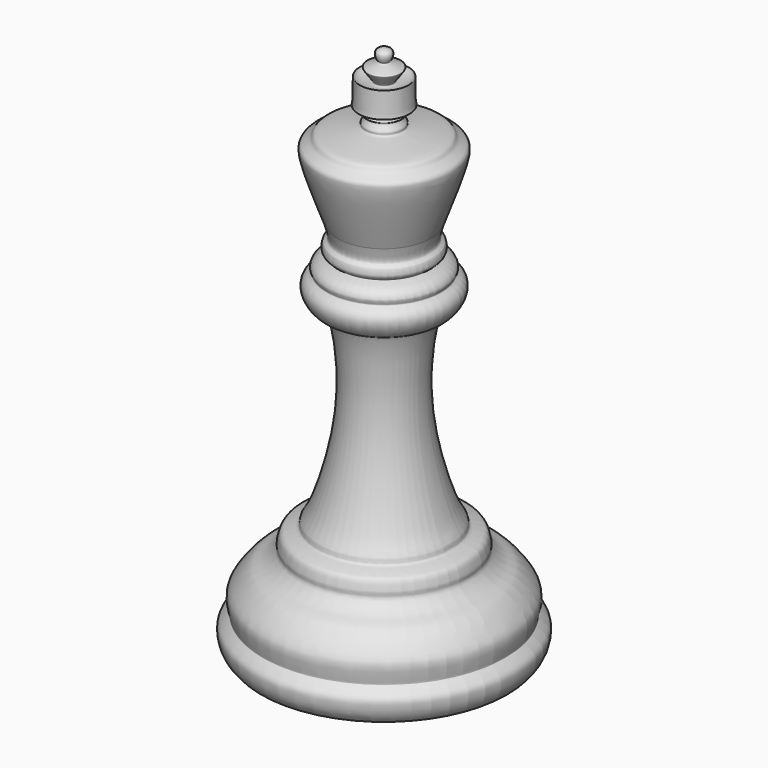
from build123d import *


with BuildPart() as f1:
    # F0 (on Front) → F1 (revolve)
    with BuildSketch(Plane.XZ):
        with BuildLine():
            add(Edge.make_bspline(
                [(5.1968609914, 11.6834519431), (6.218441868, 14.4839049359), (7.5850443695, 18.2301634584), (7.376488045, 19.3110571479), (6.2440103526, 19.7319094437), (6.3166378152, 20.557495652), (1.8331770813, 20.7960761587), (2.0893138683, 21.2951581913), (1.9862298243, 21.5611901032), (1.4972981293, 22.1288291381), (2.1007020544, 22.2621416821), (1.926576114, 22.6142654309), (0.8062071213, 24.1069602548), (2.9751149831, 22.8016434673), (2.6382284802, 23.4175411427), (2.7705577066, 26.2855445539), (2.6045340645, 25.4175150798), (0.8885045581, 25.1216459342), (1.0575875606, 25.6370810941), (1.7879172578, 26.5685371018), (1.9605993627, 26.9108633673), (0.3336987308, 27.2037301503), (0.6403317968, 27.4335544658), (0.8297464052, 27.8559778982), (0.8176082704, 28.4252916602), (0.2292179278, 28.6375497874), (0.0643784667, 28.6175346415), (0, 28.6097176759)],
                knots=[0, 0, 0, 0, 0.1174938574, 0.1571754162, 0.2006753611, 0.2356574566, 0.3232093148, 0.344325419, 0.3684583762, 0.40182775, 0.4281436079, 0.4542966926, 0.4988550545, 0.5511682811, 0.5766404883, 0.6457000187, 0.668953563, 0.7229216893, 0.7461746173, 0.7954717811, 0.8162697801, 0.8672673017, 0.8847740186, 0.9152752602, 0.9466205871, 0.9791525358, 1, 1, 1, 1], degree=3))
            Line((0, 28.6097176759), (0, -30.9770032763))
            add(Edge.make_bspline(
                [(13.6192804202, -30.1207844168), (12.7748706513, -30.3135429528), (10.7916718802, -30.7662597568), (5.6477105328, -30.8654461447), (1.9222300495, -30.939034179), (0, -30.9770032763)],
                knots=[0, 0, 0, 0, 0.2641152779, 0.6203067679, 1, 1, 1, 1], degree=3))
            add(Edge.make_bspline(
                [(13.6192804202, -30.1207844168), (14.0759363035, -29.661282589), (14.4034380415, -28.9151717879), (14.5048240934, -28.0151077029), (14.3669138982, -27.375895914), (13.4778633215, -26.6536462862), (13.3564997979, -26.6119397358), (13.6187476305, -25.7140412444), (13.7029087093, -24.6097291855), (13.2109349613, -23.6866553727), (11.6597215515, -21.7573959567), (10.5235456228, -21.7231516253), (9.0996828166, -20.3584377316), (9.3896076459, -19.8958965991), (9.1645984131, -19.0260751314), (8.8983861995, -18.3258447437), (7.2478860761, -18.2212913183), (7.3856744392, -17.4467526555), (6.5020368794, -16.5625369451), (4.5673856579, -10.2970587605), (3.9105598077, -4.2805955629), (4.358698749, 0.7051251264), (4.9419834188, 2.8555241992), (5.1411936136, 3.2304857959), (6.0264755867, 3.3553821363), (6.6684379827, 3.9258082304), (7.2202126264, 4.7885664194), (7.320393564, 5.8324876696), (6.7347106829, 6.5227751887), (6.1635163374, 6.6934786898), (6.4668189704, 7.0818367844), (6.3889100631, 7.6028903634), (5.6305591752, 8.3105421829), (4.7298017985, 8.4038710136), (5.1503781366, 8.6333181802), (5.4586207499, 8.9804270299), (5.4306981213, 9.3604516737), (5.3298387623, 9.9178926203), (4.7002850439, 10.0166552476), (4.9983378177, 11.017093108), (5.1968609914, 11.6834519431)],
                knots=[0.1421138956, 0.1421138956, 0.1421138956, 0.1421138956, 0.1690606862, 0.1890445407, 0.2072082126, 0.2300497852, 0.2366320697, 0.2567034759, 0.2801838693, 0.303004198, 0.3365674829, 0.3608934582, 0.3896051506, 0.4042477708, 0.4244632188, 0.4431526941, 0.4690213789, 0.4848944007, 0.5075867486, 0.5631053568, 0.619978695, 0.6694844516, 0.7006657488, 0.7135294128, 0.7333335058, 0.753904354, 0.776100807, 0.798052295, 0.8186239744, 0.8333392374, 0.8462639604, 0.8615614762, 0.8844393371, 0.9021087832, 0.9135024664, 0.9286508631, 0.9421996255, 0.9579209521, 0.9719725268, 1, 1, 1, 1], degree=3))
        make_face()
    revolve(axis=Axis((0, 0, -2.3902823241), (0, 0, -1)))


solid = f1.part
